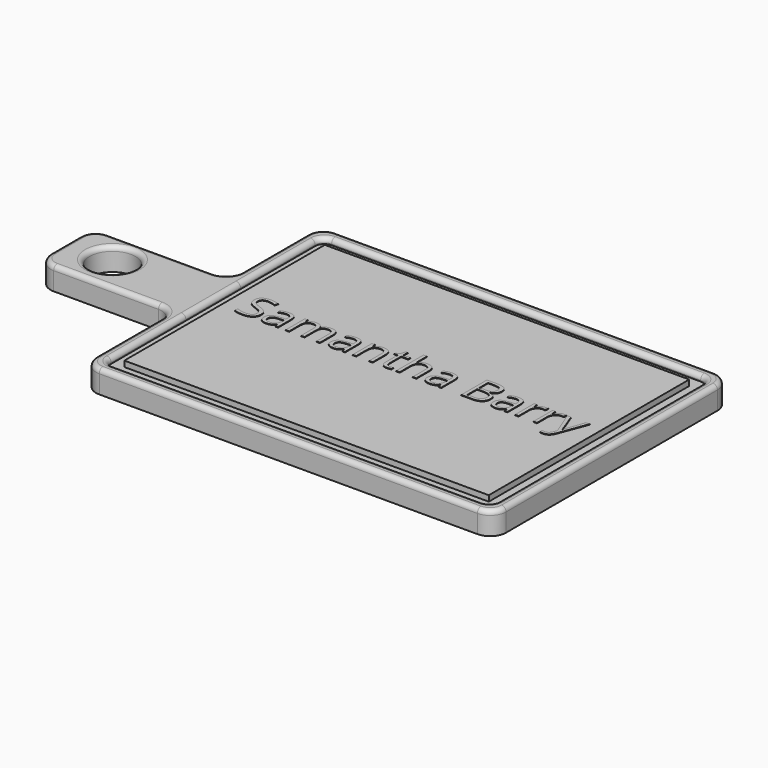
from build123d import *

# Parameters (mm, degrees)
F0_W         = 152.4
F0_H         = 76.2
F1_DEPTH     = 25.4
F2_R         = 25.4
F3_DEPTH     = 25.4
F5_DEPTH     = 6.35
F6_R         = 10.16
F7_R         = 17.78
F8_R         = 5.07999
F9_TEXT_SIZE = 50.2897683915
F10_DEPTH    = 0.508


# Not quite as in the source:
# - a fillet or chamfer is up to 0.001 mm smaller than in the source, because OpenCascade refuses the exact size
# - ends of sketch curves that miss each other by under 0.0002 mm in the source are joined
# - Text() gives the source's letters only with a copy of the font that has no kerning and outlines rounded to 1/6400 em; it was checked with that copy


with BuildPart() as f1:
    # F0 (on Top) → F1 (new body)
    with BuildSketch(Plane.XY):
        Polygon((0, 127), (0, 0), (457.2, 0), (457.2, 330.2), (0, 330.2), (0, 203.2), align=None)
        with Locations((-76.2, 165.1)):
            Rectangle(F0_W, F0_H)
    extrude(amount=F1_DEPTH)

    # F2 (on face) → F3 (cut)
    with BuildSketch(Plane.XY.offset(25.4)):
        with Locations((-101.6, 167.64)):
            Circle(F2_R)
    extrude(amount=-F3_DEPTH, mode=Mode.SUBTRACT)

    # F4 (on face) → F5 (cut)
    with BuildSketch(Plane.XY.offset(25.4)):
        Polygon((12.6999998465, 317.5000001535), (12.6999998465, 203.2), (12.7000047684, 127), (12.6999998465, 12.6999998465), (444.5000001535, 12.6999998465), (444.5000001535, 317.5000001535), align=None)
        Polygon((25.399996233, 127), (25.399996233, 203.2), (25.399996233, 304.800003767), (431.800003767, 304.800003767), (431.800003767, 25.399996233), (25.399996233, 25.399996233), align=None, mode=Mode.SUBTRACT)
    extrude(amount=-F5_DEPTH, mode=Mode.SUBTRACT)

    # F6
    f6_edges = [f1.edges().sort_by_distance(p)[0] for p in [
        (12.7, 317.5, 22.225),
        (12.7, 12.7, 22.225),
        (444.5, 12.7, 22.225),
        (444.5, 317.5, 22.225),
    ]]
    fillet(f6_edges, radius=F6_R)

    # F7
    f7_edges = [f1.edges().sort_by_distance(p)[0] for p in [
        (0, 0, 12.7),
        (0, 127, 12.7),
        (-152.4, 127, 12.7),
        (-152.4, 203.2, 12.7),
        (0, 203.2, 12.7),
        (0, 330.2, 12.7),
        (457.2, 330.2, 12.7),
        (457.2, 0, 12.7),
    ]]
    fillet(f7_edges, radius=F7_R)

    # F8 (radius 5.08 in the source; OpenCascade refuses exactly that, so slightly less here)
    f8_edges = [f1.edges().sort_by_distance(p)[0] for p in [
        (0, 63.5, 25.4),
        (-5.207641, 121.792359, 25.4),
        (5.207641, 5.207641, 25.4),
        (-76.2, 127, 25.4),
        (228.6, 0, 25.4),
        (-147.192359, 132.207641, 25.4),
        (451.992359, 5.207641, 25.4),
        (-152.4, 165.1, 25.4),
        (457.2, 165.1, 25.4),
        (-147.192359, 197.992359, 25.4),
        (451.992359, 324.992359, 25.4),
        (-76.2, 203.2, 25.4),
        (228.6, 330.2, 25.4),
        (-5.207641, 208.407641, 25.4),
        (5.207641, 324.992359, 25.4),
        (0, 266.7, 25.4),
        (12.7, 255.27, 25.4),
        (15.675795, 314.524205, 25.4),
        (12.700002, 165.1, 25.4),
        (228.6, 317.5, 25.4),
        (12.700003, 74.93, 25.4),
        (441.524205, 314.524205, 25.4),
        (15.675795, 15.675795, 25.4),
        (444.5, 165.1, 25.4),
        (228.6, 12.7, 25.4),
        (441.524205, 15.675795, 25.4),
        (-127, 167.64, 25.4),
    ]]
    fillet(f8_edges, radius=F8_R)

    # F9 (on face) → F10 (join)
    with BuildSketch(Plane.XY.offset(25.4)):
        with Locations((39.6505065179, 157.4030283698)):
            Text('Samantha Barry', F9_TEXT_SIZE, font='Open Sans', text_align=(TextAlign.LEFT, TextAlign.BOTTOM))
    extrude(amount=F10_DEPTH)


solid = f1.part
